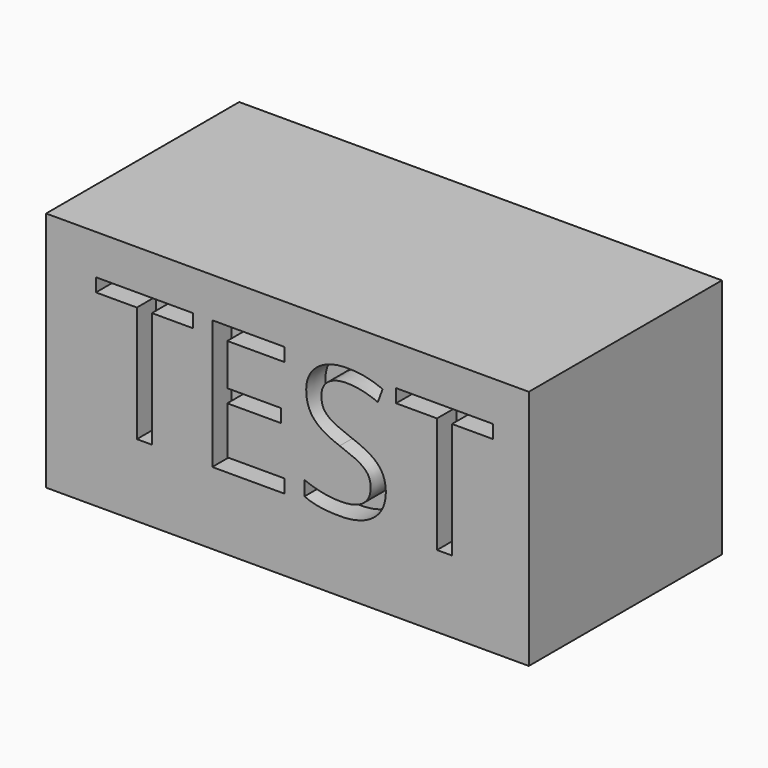
from build123d import *

# Parameters (mm, degrees)
F0_W         = 50.8
F0_H         = 25.4
F1_DEPTH     = 25.4
F2_TEXT_SIZE = 19.0469363843
F3_DEPTH     = 2.54
F4_TEXT_SIZE = 10.1490052443
F5_DEPTH     = 2.54


# Not quite as in the source:
# - Text() gives the source's letters only with a copy of the font that has no kerning and outlines rounded to 1/6400 em; it was checked with that copy


with BuildPart() as f1:
    # F0 (on Top) → F1 (new body)
    with BuildSketch(Plane.XY):
        Rectangle(F0_W, F0_H)
    extrude(amount=F1_DEPTH)

    # F2 (on face) → F3 (cut)
    with BuildSketch(Plane.XZ.offset(12.7)):
        with Locations((-20.32, 7.6005564258)):
            Text('TEST', F2_TEXT_SIZE, font='Open Sans', text_align=(TextAlign.LEFT, TextAlign.BOTTOM))
    extrude(amount=-F3_DEPTH, mode=Mode.SUBTRACT)

    # F4 (on face) → F5 (cut)
    with BuildSketch(Plane(origin=(0, 12.7, 0), x_dir=(-1, 0, 0), z_dir=(0, 1, 0))):
        with Locations((-17.6588834922, 8.1002190305)):
            Text('12.7MM', F4_TEXT_SIZE, font='Open Sans', text_align=(TextAlign.LEFT, TextAlign.BOTTOM))
    extrude(amount=-F5_DEPTH, mode=Mode.SUBTRACT)


solid = f1.part
